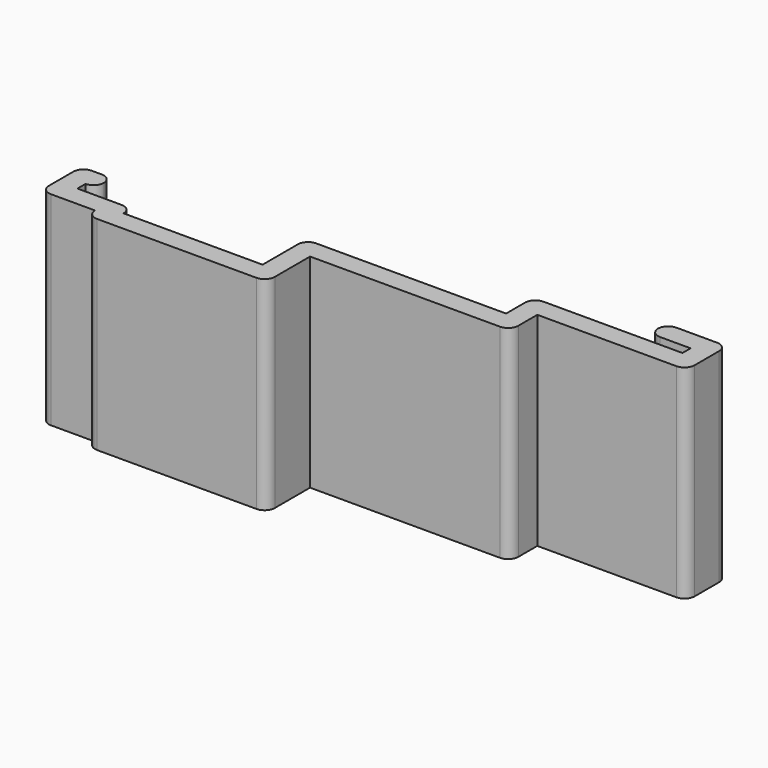
from build123d import *

# Parameters (mm, degrees)
F1_DEPTH = 30
F2_R     = 1.49999


# Not quite as in the source:
# - a fillet or chamfer is up to 0.001 mm smaller than in the source, because OpenCascade refuses the exact size


with BuildPart() as f1:
    # F0 (on Top) → F1 (new body)
    with BuildSketch(Plane.XY):
        Polygon((0, 8), (0, 0), (-20.5, 0), (-20.5, 1.5), (-28.5, 1.5), (-28.5, 3), (-27, 3), (-27, 6), (-31.5, 6), (-31.5, -1.5), (-23.5, -1.5), (-23.5, -3), (3, -3), (3, 5), (32.5, 5), (32.5, 10), (54.5, 10), (54.5, 17.5), (45.5, 17.5), (45.5, 14.5), (51.5, 14.5), (51.5, 13), (29.5, 13), (29.5, 8), align=None)
    extrude(amount=F1_DEPTH)

    # F2 (radius 1.5 in the source; OpenCascade refuses exactly that, so slightly less here)
    f2_edges = [f1.edges().sort_by_distance(p)[0] for p in [
        (-23.5, -3, 15),
        (-31.5, -1.5, 15),
        (-20.5, 1.5, 15),
        (-27, 6, 15),
        (-27, 3, 15),
        (-31.5, 6, 15),
        (3, -3, 15),
        (0, 8, 15),
        (32.5, 5, 15),
        (29.5, 13, 15),
        (45.5, 17.5, 15),
        (45.5, 14.5, 15),
        (54.5, 10, 15),
        (54.5, 17.5, 15),
    ]]
    fillet(f2_edges, radius=F2_R)


solid = f1.part
